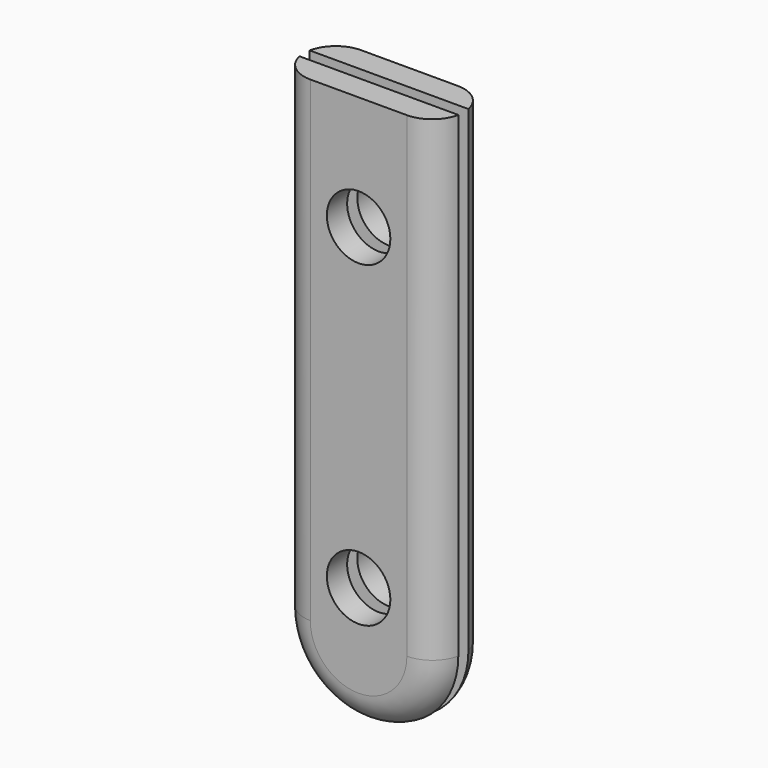
from build123d import *

# Parameters (mm, degrees)
F1_DEPTH    = 2.032
F2_R        = 2.54
F3_DEPTH    = 2.032
F4_T1_DEPTH = 44.3217039467
F4_T4_ANGLE = 180


# Not quite as in the source:
# - a fillet or chamfer that OpenCascade refuses, or shapes differently, is made with other operations: its cross-section is extruded or revolved along the edge and cut away or added


with BuildPart() as f1:
    # F0 (on Front) → F1 (new body)
    with BuildSketch(Plane.XZ):
        with BuildLine():
            Line((12.7, 25.0395175091), (0, 25.0395175091))
            Line((0, 25.0395175091), (0, -13.0604824909))
            ThreePointArc((0, -13.0604824909), (1.8598719395, -17.5506105514), (6.35, -19.4104824909))
            ThreePointArc((6.35, -19.4104824909), (10.8401280605, -17.5506105514), (12.7, -13.0604824909))
            Line((12.7, -13.0604824909), (12.7, 25.0395175091))
        make_face()
    extrude(amount=F1_DEPTH)

    # F2 (on face) → F3 (cut)
    with BuildSketch(Plane.XZ.offset(2.032)):
        with Locations((6.35, -9.5044824909)):
            Circle(F2_R)
        with Locations((6.35, 15.8955175091)):
            Circle(F2_R)
    extrude(amount=-F3_DEPTH, mode=Mode.SUBTRACT)

    # F4: fillet of radius 2.54 on 1 edges, made by hand

    # F4_s2 → F4_t1 (cut)
    with BuildSketch(Plane.XY.offset(-13.0604824909)):
        with BuildLine():
            ThreePointArc((12.7, 0), (11.8177554727, -1.4594755399), (10.2113184213, -2.032))
            Line((10.2113184213, -2.032), (12.7, -2.032))
            Line((12.7, -2.032), (12.7, 0))
        make_face()
        with BuildLine():
            ThreePointArc((0, 0), (0.8822445273, -1.4594755399), (2.4886815787, -2.032))
            Line((2.4886815787, -2.032), (0, -2.032))
            Line((0, -2.032), (0, 0))
        make_face()
    extrude(amount=F4_T1_DEPTH, mode=Mode.SUBTRACT)

    # F4_s3 → F4_t4 (revolve, cut)
    with BuildSketch(Plane.XY.offset(-13.0604824909)):
        with BuildLine():
            ThreePointArc((12.7, 0), (11.8177554727, -1.4594755399), (10.2113184213, -2.032))
            Line((10.2113184213, -2.032), (12.7, -2.032))
            Line((12.7, -2.032), (12.7, 0))
        make_face()
    revolve(axis=Axis((6.35, -2.032, -13.0604824909), (0, 1, 0)), revolution_arc=F4_T4_ANGLE, mode=Mode.SUBTRACT)


with BuildPart() as f6_1:
    # F6: instance of F1
    add(f1.part.mirror(Plane(origin=(6.35, 0.508, 3.4947340596), x_dir=(1, 0, 0), z_dir=(0, 1, 0))))


solid = Compound([f1.part, f6_1.part])
